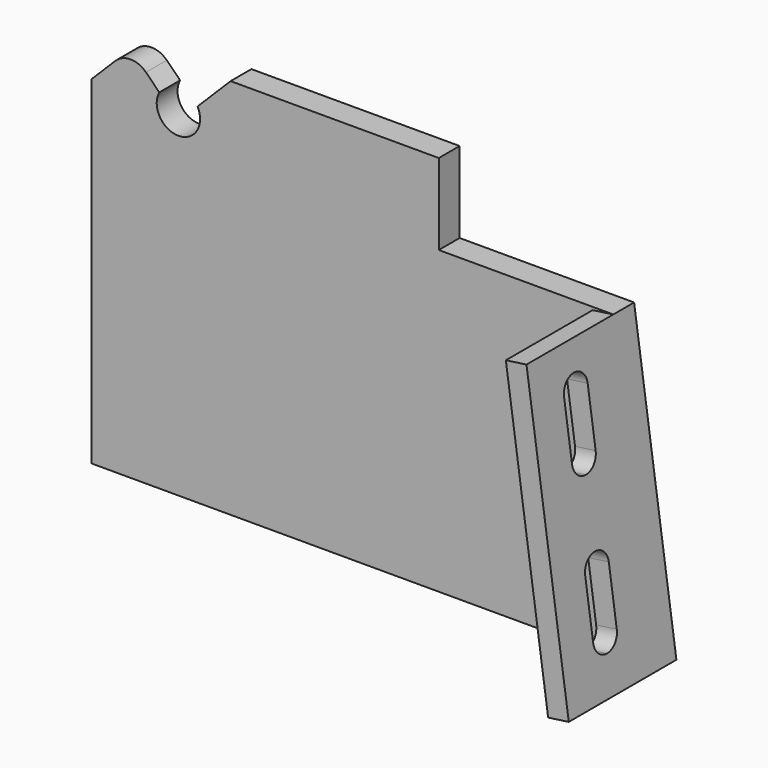
from build123d import *

# Parameters (mm, degrees)
F1_DEPTH  = 15.875
F2_W      = 4.318
F2_H      = 12.7
F3_DEPTH  = 9.175040233
F4_R      = 2.15899
F5_R      = 3.175
F6_DEPTH  = 3.81
F8_DEPTH  = 25.4
F10_DEPTH = 25.4
F11_R     = 3.175


# Not quite as in the source:
# - a fillet or chamfer is up to 0.001 mm smaller than in the source, because OpenCascade refuses the exact size


with BuildPart() as f1:
    # F0 (on Front) → F1 (new body)
    with BuildSketch(Plane.XZ):
        Polygon((9.2045814112, -87.6168819653), (3.0183370735, -43.5994663098), (0, -44.0236659215), (6.1862443377, -88.041081577), align=None)
    extrude(amount=F1_DEPTH)

    # F2 (on face) → F3 (cut, through all)
    with BuildSketch(Plane(origin=(-6.067283434, 0, -0.8527010782), x_dir=(0, -1, 0), z_dir=(-0.9902680687, 0, -0.139173101))):
        with Locations((7.9375, -54.072730631)):
            Rectangle(F2_W, F2_H)
        with Locations((7.9375, -76.297730631)):
            Rectangle(F2_W, F2_H)
    extrude(amount=-F3_DEPTH, mode=Mode.SUBTRACT)

    # F4 (radius 2.159 in the source; OpenCascade refuses exactly that, so slightly less here)
    f4_edges = [f1.edges().sort_by_distance(p)[0] for p in [
        (2.083606, -5.7785, -47.898898),
        (5.176728, -5.7785, -69.907605),
        (5.176728, -10.0965, -69.907605),
        (2.083606, -10.0965, -47.898898),
        (3.851104, -10.0965, -60.475302),
        (6.944226, -10.0965, -82.48401),
        (6.944226, -5.7785, -82.48401),
        (3.851104, -5.7785, -60.475302),
    ]]
    fillet(f4_edges, radius=F4_R)

    # F5 (on Front) → F6 (join)
    with BuildSketch(Plane.XZ):
        Polygon((9.2045814112, -87.6168819653), (3.0183370735, -43.5994663098), (-22.5109767612, -43.5994663098), (-22.5109767612, -25.4), (-73.3109767612, -25.4), (-73.3109767612, -87.6168819653), align=None)
        with Locations((-60.6109767612, -38.1)):
            Circle(F5_R, mode=Mode.SUBTRACT)
    extrude(amount=-F6_DEPTH)

    # F7 (on Front) → F8 (cut)
    with BuildSketch(Plane.XZ):
        Polygon((-73.3109767612, -38.1), (-60.6109767612, -25.4), (-73.3109767612, -25.4), align=None)
    extrude(amount=-F8_DEPTH, mode=Mode.SUBTRACT)

    # F9 (on Front) → F10 (cut)
    with BuildSketch(Plane.XZ):
        Polygon((-74.5969353161, -25.4), (-60.6109767612, -39.3859585549), (-52.9750182062, -31.75), (-22.5109767612, -31.75), (-22.5109767612, -25.4), align=None)
    extrude(amount=-F10_DEPTH, mode=Mode.SUBTRACT)

    # F11
    f11_edges = [f1.edges().sort_by_distance(p)[0] for p in [
        (-67.603956, 1.905, -32.392979),
    ]]
    fillet(f11_edges, radius=F11_R)


solid = f1.part
